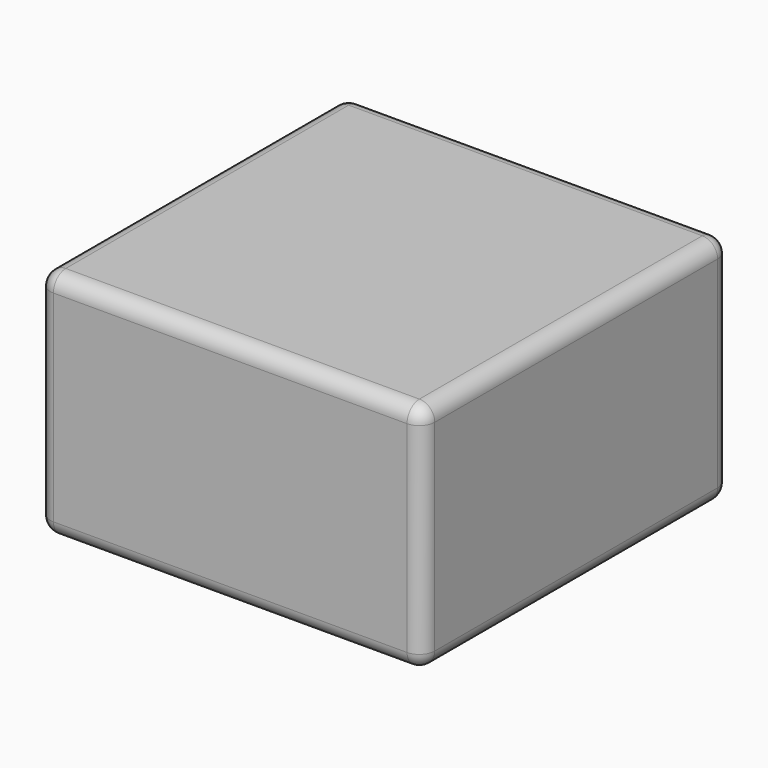
from build123d import *

# Parameters (mm, degrees)
F0_W          = 31.75
F0_H          = 31.75
F5_DEPTH      = 19.177
F1_W          = 28.575
F1_H          = 28.575
F6_DEPTH      = 18.161
F6_DEPTH_BACK = 0.381
F2_R          = 6.5405
F7_DEPTH      = 15.875
F3_R          = 5.461
F8_DEPTH      = 15.875
F8_DEPTH_BACK = 0.635
F4_W          = 1.016
F4_H          = 2.286
F10_DEPTH     = 17.526
F15_ANGLE     = 90
F16_R         = 1.26999


# Not quite as in the source:
# - a fillet or chamfer is up to 0.001 mm smaller than in the source, because OpenCascade refuses the exact size


with BuildPart() as f5:
    # F0 (on Top) → F5 (new body)
    with BuildSketch(Plane.XY):
        with Locations((0, -0.3175)):
            Rectangle(F0_W, F0_H)
    extrude(amount=F5_DEPTH)

    # F1 (on face) → F6 (cut, two sides)
    with BuildSketch(Plane.XY) as f6_sk:
        Rectangle(F1_W, F1_H)
    extrude(amount=F6_DEPTH, mode=Mode.SUBTRACT)
    extrude(f6_sk.sketch, amount=-F6_DEPTH_BACK, mode=Mode.SUBTRACT)

    # F16 (radius 1.27 in the source; OpenCascade refuses exactly that, so slightly less here)
    f16_edges = [f5.edges().sort_by_distance(p)[0] for p in [
        (0, -16.1925, 19.177),
        (-15.875, -0.3175, 19.177),
        (0, 15.5575, 19.177),
        (15.875, -0.3175, 19.177),
        (-15.875, -16.1925, 9.5885),
        (15.875, -16.1925, 9.5885),
        (-15.875, 15.5575, 9.5885),
        (15.875, 15.5575, 9.5885),
        (15.875, -0.3175, 0),
        (0, -16.1925, 0),
        (-15.875, -0.3175, 0),
        (0, 15.5575, 0),
    ]]
    fillet(f16_edges, radius=F16_R)


with BuildPart() as f7:
    # F2 (on face) → F7 (new body)
    with BuildSketch(Plane.XY):
        Circle(F2_R)
    extrude(amount=F7_DEPTH)

    # F3 (on face) → F8 (cut, two sides)
    with BuildSketch(Plane.XY) as f8_sk:
        Circle(F3_R)
    extrude(amount=F8_DEPTH, mode=Mode.SUBTRACT)
    extrude(f8_sk.sketch, amount=-F8_DEPTH_BACK, mode=Mode.SUBTRACT)


with BuildPart() as f7_1:
    # F9: moved
    add(f7.part.moved(Location((0, 0, 2.286))))


with BuildPart() as f10:
    # F4 (on face) → F10 (new body)
    with BuildSketch(Plane.XY):
        with Locations((0, -0.357)):
            Rectangle(F4_W, F4_H)
    extrude(amount=F10_DEPTH)


with BuildPart() as f10_1:
    # F11: moved
    add(f10.part.moved(Location((8.0645, 13.8557, 0.635))))


with BuildPart() as f12_1:
    # F12: instance of F10
    add(f10_1.part.mirror(Plane.XZ))


with BuildPart() as f13_1:
    # F13: instance of F12_1
    add(f12_1.part.mirror(Plane.YZ))


with BuildPart() as f13_2:
    # F13: instance of F10
    add(f10_1.part.mirror(Plane.YZ))


with BuildPart() as f15_1:
    # F15: copy of F12_1
    add(f12_1.part.rotate(Axis((0, 0, 4.273429513), (0, 0, -1)), F15_ANGLE))


with BuildPart() as f15_2:
    # F15: copy of F13_1
    add(f13_1.part.rotate(Axis((0, 0, 4.273429513), (0, 0, -1)), F15_ANGLE))


with BuildPart() as f15_3:
    # F15: copy of F10
    add(f10_1.part.rotate(Axis((0, 0, 4.273429513), (0, 0, -1)), F15_ANGLE))


with BuildPart() as f15_4:
    # F15: copy of F13_2
    add(f13_2.part.rotate(Axis((0, 0, 4.273429513), (0, 0, -1)), F15_ANGLE))


solid = Compound([f5.part, f7_1.part, f10_1.part, f12_1.part, f13_1.part, f13_2.part, f15_1.part, f15_2.part, f15_3.part, f15_4.part])
